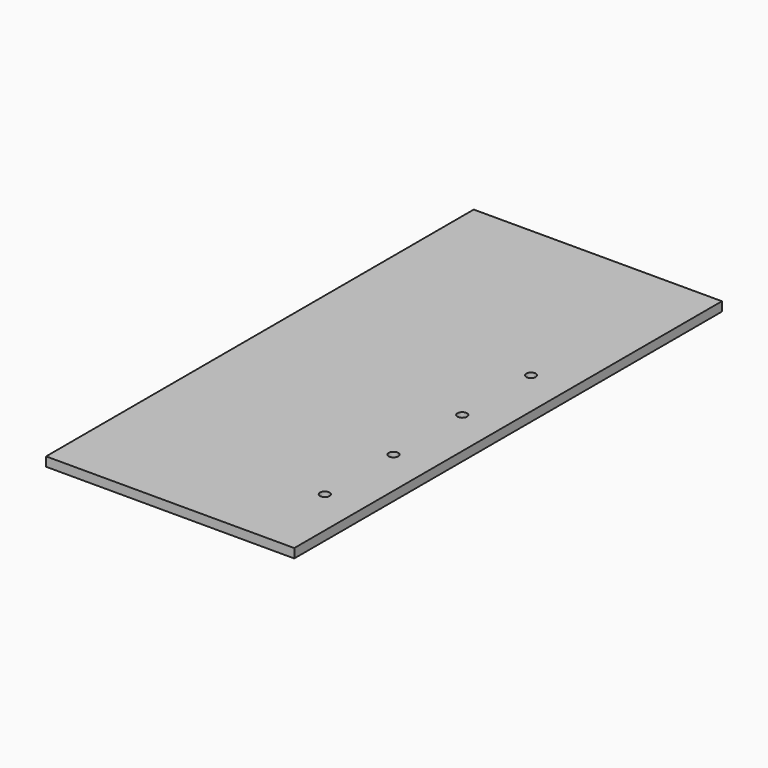
from build123d import *

# Parameters (mm, degrees)
F0_W     = 82.55
F0_H     = 177.8
F1_DEPTH = 3.048
F2_R     = 1.5875
F3_DEPTH = 25.4


# Not quite as in the source:
# - a feature names something its author has since deleted; it is built from what else it names


with BuildPart() as f1:
    # F0 (on Top) → F1 (new body)
    with BuildSketch(Plane.XY):
        Rectangle(F0_W, F0_H)
    extrude(amount=F1_DEPTH)

    # F2 (on face) → F3 (cut)
    with BuildSketch(Plane.XY.offset(3.048)):
        with Locations((28.575, 25.4)):
            Circle(F2_R)
        with Locations((28.575, -3.175)):
            Circle(F2_R)
        with Locations((28.575, -31.75)):
            Circle(F2_R)
        with Locations((28.575, -60.325)):
            Circle(F2_R)
    extrude(amount=-F3_DEPTH, mode=Mode.SUBTRACT)


solid = f1.part
